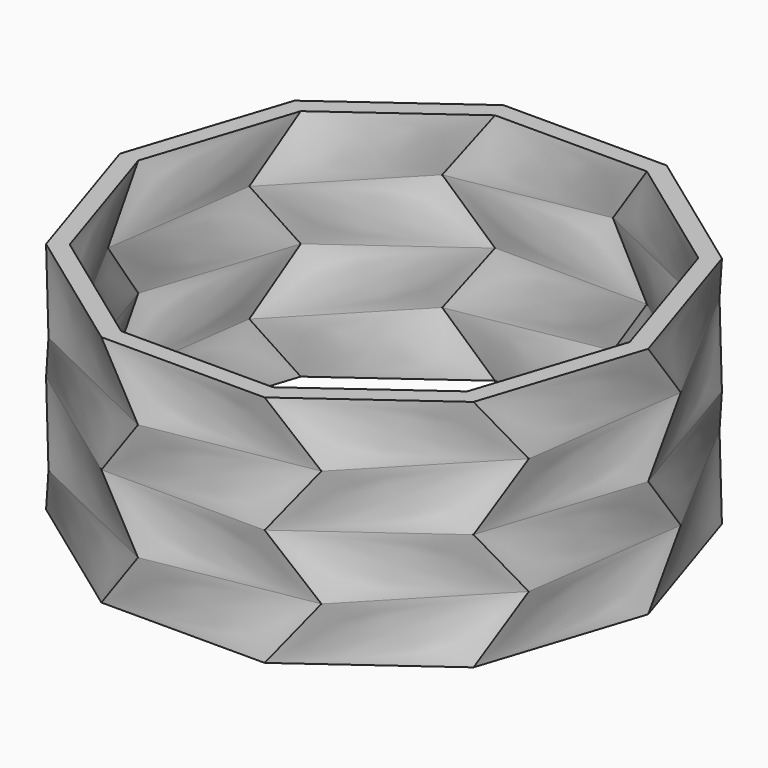
from build123d import *


with BuildPart() as f5:
    # F0 (on Top) → F5 section 0
    with BuildSketch(Plane.XY):
        Polygon((12.9967878493, 40), (-12.9967878493, 40), (-34.0260323341, 24.72135955), (-42.0584889695, 0), (-34.0260323341, -24.72135955), (-12.9967878493, -40), (12.9967878493, -40), (34.0260323341, -24.72135955), (42.0584889695, 0), (34.0260323341, 24.72135955), align=None)
    # F3 (on offset) → F5 section 1
    with BuildSketch(Plane.XY.offset(10)):
        Polygon((-29.2162814115, -30.2543450579), (-5.8534103316, -41.649178646), (19.7452645449, -37.1354415949), (37.8019194822, -18.4372280418), (41.4195260172, 7.303379965), (29.2162814115, 30.2543450579), (5.8534103316, 41.649178646), (-19.7452645449, 37.1354415949), (-37.8019194822, 18.4372280418), (-41.4195260172, -7.303379965), align=None)
    loft()


with BuildPart() as f6:
    # F1 (on Top) → F6 section 0
    with BuildSketch(Plane.XY):
        Polygon((-13.971546938, 43), (-36.5779847591, 26.5754615162), (-45.2128756422, 0), (-36.5779847591, -26.5754615162), (-13.971546938, -43), (13.971546938, -43), (36.5779847591, -26.5754615162), (45.2128756422, 0), (36.5779847591, 26.5754615162), (13.971546938, 43), align=None)
    # F4 (on offset) → F6 section 1
    with BuildSketch(Plane.XY.offset(10)):
        Polygon((-21.2261593858, 39.9205997146), (-40.6370634433, 19.8200201449), (-44.5259904685, -7.8511334624), (-31.4075025174, -32.5234209372), (-6.2924161065, -44.7728670445), (21.2261593858, -39.9205997146), (40.6370634433, -19.8200201449), (44.5259904685, 7.8511334624), (31.4075025174, 32.5234209372), (6.2924161065, 44.7728670445), align=None)
    loft()

    # F7: cut F5
    add(f5.part, mode=Mode.SUBTRACT)

    # F11 (on face) → F14 section 0
    with BuildSketch(Plane.XY.offset(10)):
        Polygon((-44.5259904685, -7.8511334624), (-31.4075025174, -32.5234209372), (-6.2924161065, -44.7728670445), (21.2261593858, -39.9205997146), (40.6370634433, -19.8200201449), (44.5259904685, 7.8511334624), (31.4075025174, 32.5234209372), (6.2924161065, 44.7728670445), (-21.2261593858, 39.9205997146), (-40.6370634433, 19.8200201449), align=None)
    # F10 (on offset) → F14 section 1
    with BuildSketch(Plane.XY.offset(20)):
        Polygon((-13.971546938, 43), (-36.5779847591, 26.5754615162), (-45.2128756422, 0), (-36.5779847591, -26.5754615162), (-13.971546938, -43), (13.971546938, -43), (36.5779847591, -26.5754615162), (45.2128756422, 0), (36.5779847591, 26.5754615162), (13.971546938, 43), align=None)
    loft()


with BuildPart() as f13:
    # F12 (on offset) → F13 section 0
    with BuildSketch(Plane.XY.offset(10)):
        Polygon((-19.7452645449, 37.1354415949), (-37.8019194822, 18.4372280418), (-41.4195260172, -7.303379965), (-29.2162814115, -30.2543450579), (-5.8534103316, -41.649178646), (19.7452645449, -37.1354415949), (37.8019194822, -18.4372280418), (41.4195260172, 7.303379965), (29.2162814115, 30.2543450579), (5.8534103316, 41.649178646), align=None)
    # F9 (on offset) → F13 section 1
    with BuildSketch(Plane.XY.offset(20)):
        Polygon((12.9967878493, 40), (-12.9967878493, 40), (-34.0260323341, 24.72135955), (-42.0584889695, 0), (-34.0260323341, -24.72135955), (-12.9967878493, -40), (12.9967878493, -40), (34.0260323341, -24.72135955), (42.0584889695, 0), (34.0260323341, 24.72135955), align=None)
    loft()


with BuildPart() as f6_1:
    add(f6.part)

    # F15: cut F13
    add(f13.part, mode=Mode.SUBTRACT)

    # F16: F6 across face


with BuildPart() as f6_2:
    add(f6_1.part)
    add(f6_1.part.mirror(Plane.XY.offset(20)))


solid = f6_2.part
